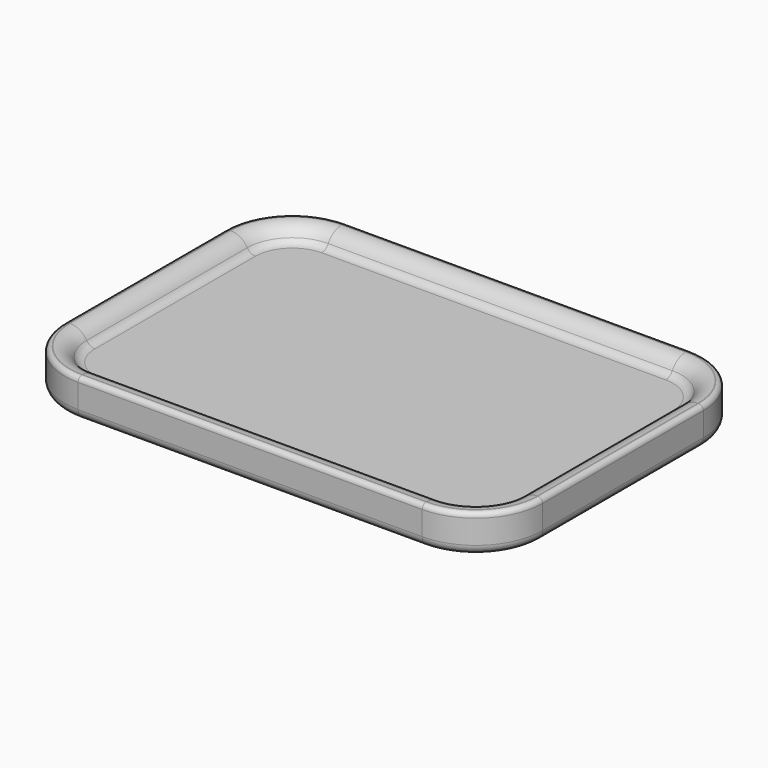
from build123d import *

# Parameters (mm, degrees)
F1_DEPTH     = 4
F2_R         = 1
F3_T         = -2.5
F4_T1_DEPTH  = 36
F4_T3_DEPTH  = 21
F4_T6_ANGLE  = 90
F4_T8_ANGLE  = 90
F4_T10_ANGLE = 90
F4_T12_ANGLE = 90
F5_R         = 1
F6_R         = 0.5
F7_R         = 2.15
F8_DEPTH     = 1.6


# Not quite as in the source:
# - a fillet or chamfer that OpenCascade refuses, or shapes differently, is made with other operations: its cross-section is extruded or revolved along the edge and cut away or added


with BuildPart() as f1:
    # F0 (on Top) → F1 (new body)
    with BuildSketch(Plane.XY):
        with BuildLine():
            Line((-18, -17.5), (18, -17.5))
            ThreePointArc((18, -17.5), (22.9497474683, -15.4497474683), (25, -10.5))
            Line((25, -10.5), (25, 10.5))
            ThreePointArc((25, 10.5), (22.9497474683, 15.4497474683), (18, 17.5))
            Line((18, 17.5), (-18, 17.5))
            ThreePointArc((-18, 17.5), (-22.9497474683, 15.4497474683), (-25, 10.5))
            Line((-25, 10.5), (-25, -10.5))
            ThreePointArc((-25, -10.5), (-22.9497474683, -15.4497474683), (-18, -17.5))
        make_face()
    extrude(amount=F1_DEPTH)

    # F2
    f2_edges = [f1.edges().sort_by_distance(p)[0] for p in [
        (0, -17.5, 0),
    ]]
    fillet(f2_edges, radius=F2_R)

    # F3
    f3_openings = [f1.faces().sort_by_distance(p)[0] for p in [
        (0, 0, 4),
    ]]
    offset(amount=F3_T, openings=f3_openings)

    # F4: fillet of radius 2 on 1 edges, made by hand

    # F4_s2 → F4_t1 (cut)
    with BuildSketch(Plane.YZ.offset(-18)):
        with BuildLine():
            ThreePointArc((16.9364916731, 4), (15.7117468017, 3.5811388301), (15, 2.5))
            Line((15, 2.5), (15, 4))
            Line((15, 4), (16.9364916731, 4))
        make_face()
        with BuildLine():
            ThreePointArc((-16.9364916731, 4), (-15.7117468017, 3.5811388301), (-15, 2.5))
            Line((-15, 2.5), (-15, 4))
            Line((-15, 4), (-16.9364916731, 4))
        make_face()
    extrude(amount=F4_T1_DEPTH, mode=Mode.SUBTRACT)

    # F4_s4 → F4_t3 (cut)
    with BuildSketch(Plane.XZ.offset(-10.5)):
        with BuildLine():
            ThreePointArc((-24.4364916731, 4), (-23.2117468017, 3.5811388301), (-22.5, 2.5))
            Line((-22.5, 2.5), (-22.5, 4))
            Line((-22.5, 4), (-24.4364916731, 4))
        make_face()
        with BuildLine():
            ThreePointArc((24.4364916731, 4), (23.2117468017, 3.5811388301), (22.5, 2.5))
            Line((22.5, 2.5), (22.5, 4))
            Line((22.5, 4), (24.4364916731, 4))
        make_face()
    extrude(amount=F4_T3_DEPTH, mode=Mode.SUBTRACT)

    # F4_s5 → F4_t6 (revolve, cut)
    with BuildSketch(Plane.XZ.offset(-10.5)):
        with BuildLine():
            ThreePointArc((24.4364916731, 4), (23.2117468017, 3.5811388301), (22.5, 2.5))
            Line((22.5, 2.5), (22.5, 4))
            Line((22.5, 4), (24.4364916731, 4))
        make_face()
    revolve(axis=Axis((18, 10.5, 4), (0, 0, 1)), revolution_arc=F4_T6_ANGLE, mode=Mode.SUBTRACT)

    # F4_s7 → F4_t8 (revolve, cut)
    with BuildSketch(Plane.YZ.offset(-18)):
        with BuildLine():
            ThreePointArc((16.9364916731, 4), (15.7117468017, 3.5811388301), (15, 2.5))
            Line((15, 2.5), (15, 4))
            Line((15, 4), (16.9364916731, 4))
        make_face()
    revolve(axis=Axis((-18, 10.5, 4), (0, 0, 1)), revolution_arc=F4_T8_ANGLE, mode=Mode.SUBTRACT)

    # F4_s9 → F4_t10 (revolve, cut)
    with BuildSketch(Plane.XZ.offset(10.5)):
        with BuildLine():
            ThreePointArc((-24.4364916731, 4), (-23.2117468017, 3.5811388301), (-22.5, 2.5))
            Line((-22.5, 2.5), (-22.5, 4))
            Line((-22.5, 4), (-24.4364916731, 4))
        make_face()
    revolve(axis=Axis((-18, -10.5, 4), (0, 0, 1)), revolution_arc=F4_T10_ANGLE, mode=Mode.SUBTRACT)

    # F4_s11 → F4_t12 (revolve, cut)
    with BuildSketch(Plane.YZ.offset(18)):
        with BuildLine():
            ThreePointArc((-16.9364916731, 4), (-15.7117468017, 3.5811388301), (-15, 2.5))
            Line((-15, 2.5), (-15, 4))
            Line((-15, 4), (-16.9364916731, 4))
        make_face()
    revolve(axis=Axis((18, -10.5, 4), (0, 0, 1)), revolution_arc=F4_T12_ANGLE, mode=Mode.SUBTRACT)

    # F5
    f5_edges = [f1.edges().sort_by_distance(p)[0] for p in [
        (0, 15, 2.5),
        (0, -15, 2.5),
        (21.181981, -13.681981, 2.5),
        (22.5, 0, 2.5),
        (21.181981, 13.681981, 2.5),
        (-21.181981, 13.681981, 2.5),
        (-22.5, 0, 2.5),
        (-21.181981, -13.681981, 2.5),
    ]]
    fillet(f5_edges, radius=F5_R)

    # F6
    f6_edges = [f1.edges().sort_by_distance(p)[0] for p in [
        (0, -17.5, 4),
        (-22.949747, -15.449747, 4),
        (22.949747, -15.449747, 4),
        (-25, 0, 4),
        (25, 0, 4),
        (-22.949747, 15.449747, 4),
        (22.949747, 15.449747, 4),
        (0, 17.5, 4),
    ]]
    fillet(f6_edges, radius=F6_R)

    # F7 (on face) → F8 (cut)
    with BuildSketch(Plane.XY):
        with Locations((-19, -11.5)):
            Circle(F7_R)
        with Locations((19, -11.5)):
            Circle(F7_R)
        with Locations((-19, 11.5)):
            Circle(F7_R)
        with Locations((19, 11.5)):
            Circle(F7_R)
    extrude(amount=F8_DEPTH, mode=Mode.SUBTRACT)


solid = f1.part
